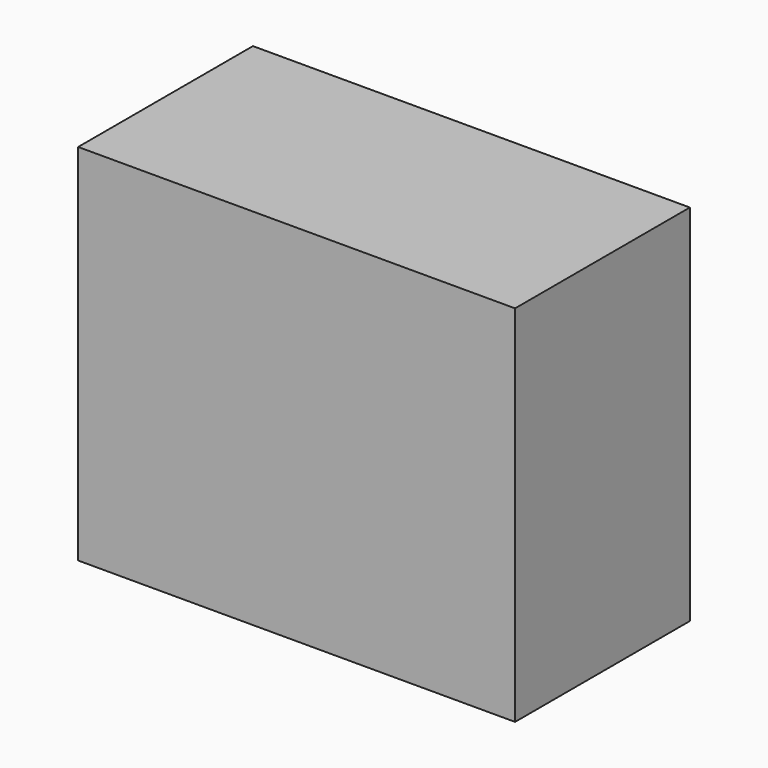
from build123d import *

# Parameters (mm, degrees)
F0_W     = 76.2
F0_H     = 63.5
F1_DEPTH = 38.1


# Not quite as in the source:
# - the program builds the solid bodies; features that only make, move or delete a surface that nothing else refers to are left out


with BuildPart() as f1:
    # F0 (on Front) → F1 (new body)
    with BuildSketch(Plane.XZ):
        Rectangle(F0_W, F0_H)
    extrude(amount=F1_DEPTH)


solid = f1.part
